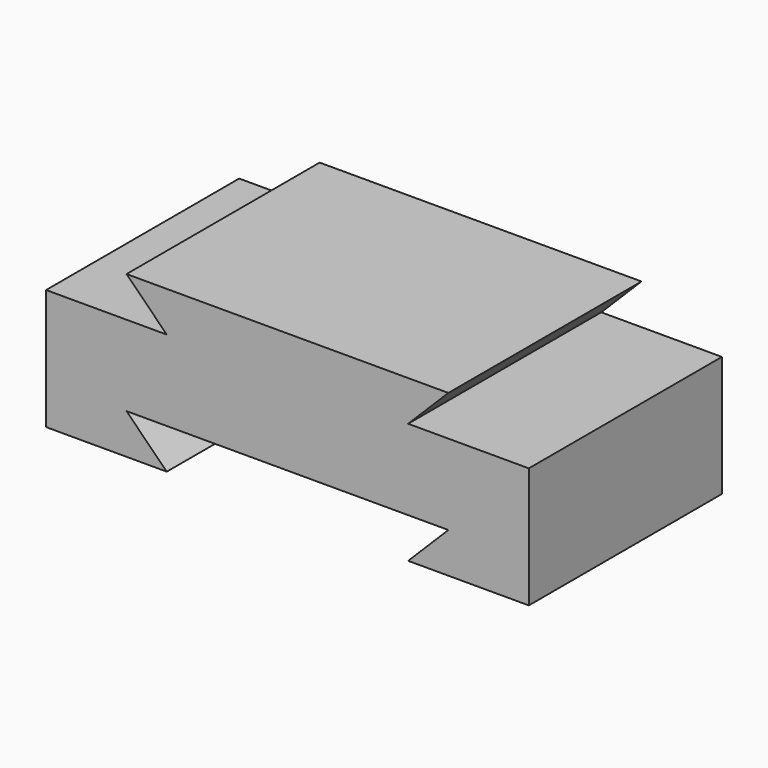
from build123d import *

# Parameters (mm, degrees)
F0_W     = 152.4
F0_H     = 76.2
F1_DEPTH = 50.8
F3_DEPTH = 76.201
F4_DEPTH = 76.201
F6_DEPTH = 76.201
F8_DEPTH = 76.201


# Not quite as in the source:
# - a feature names something its author has since deleted; it is built from what else it names


with BuildPart() as f1:
    # F0 (on Top) → F1 (new body)
    with BuildSketch(Plane.XY):
        Rectangle(F0_W, F0_H)
    extrude(amount=F1_DEPTH)

    # F2 (on face) → F3 (cut, through all)
    with BuildSketch(Plane.XZ.offset(38.1)):
        Polygon((-38.1, 0), (0, 0), (0, 12.7), (-50.8, 12.7), align=None)
    extrude(amount=-F3_DEPTH, mode=Mode.SUBTRACT)

    # F2 (on face) → F4 (cut, through all)
    with BuildSketch(Plane.XZ.offset(38.1)):
        Polygon((0, 12.7), (0, 0), (38.1, 0), (50.8, 12.7), align=None)
    extrude(amount=-F4_DEPTH, mode=Mode.SUBTRACT)

    # F5 (on face) → F6 (cut, through all)
    with BuildSketch(Plane.XZ.offset(38.1)):
        Polygon((-76.2, 38.1), (-38.1, 38.1), (-50.8, 50.8), (-76.2, 50.8), align=None)
    extrude(amount=-F6_DEPTH, mode=Mode.SUBTRACT)

    # F7 (on face) → F8 (cut, through all)
    with BuildSketch(Plane.XZ.offset(38.1)):
        Polygon((50.8, 50.8), (38.1, 38.1), (76.2, 38.1), (76.2, 50.8), align=None)
    extrude(amount=-F8_DEPTH, mode=Mode.SUBTRACT)


solid = f1.part
